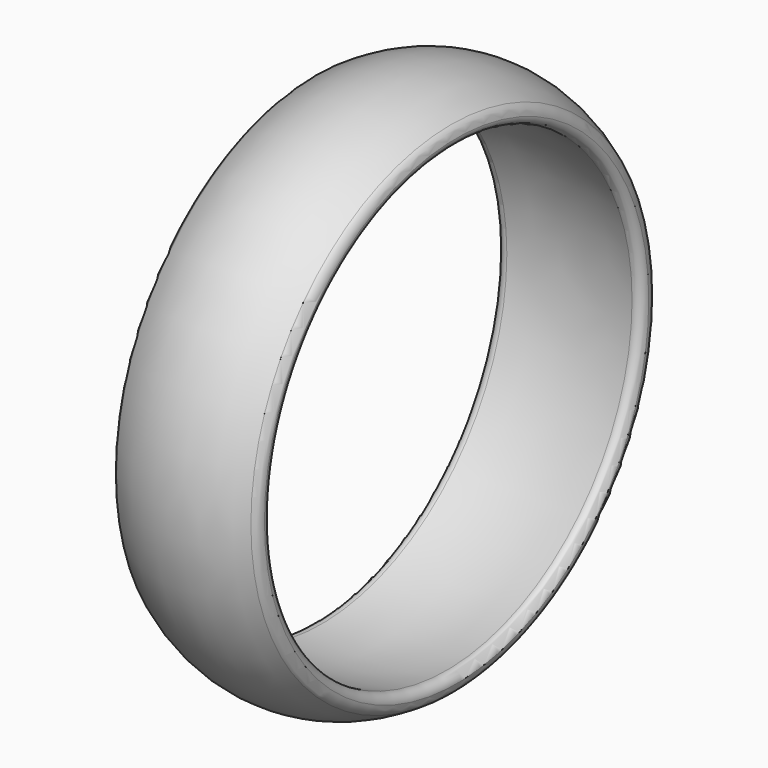
from build123d import *


# Not quite as in the source:
# - a feature names something its author has since deleted; it is built from what else it names


with BuildPart() as f1:
    # F0 (on Top) → F1 (revolve)
    with BuildSketch(Plane.XY):
        with BuildLine():
            ThreePointArc((-2.7745581576, 10.3450620873), (-2.9400449288, 10.1645927001), (-3, 9.9271891184))
            ThreePointArc((-3, 9.9271891184), (-2.8743548414, 9.6575319112), (-2.5870683925, 9.5802777102))
            ThreePointArc((-2.5870683925, 9.5802777102), (0, 9.8050593655), (2.5870683925, 9.5802777102))
            ThreePointArc((2.5870683925, 9.5802777102), (2.8743548414, 9.6575319112), (3, 9.9271891184))
            ThreePointArc((3, 9.9271891184), (2.9400449288, 10.1645927001), (2.7745581576, 10.3450620873))
            ThreePointArc((2.7745581576, 10.3450620873), (0, 11.175), (-2.7745581576, 10.3450620873))
        make_face()
    revolve(axis=Axis((2.32582842, 0, 0), (1, 0, 0)))


solid = f1.part
